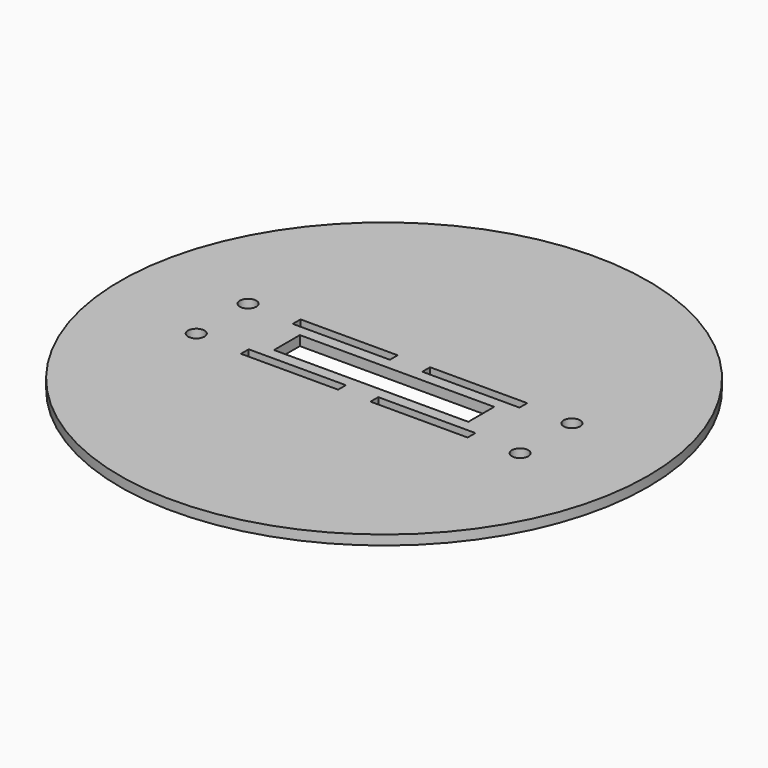
from build123d import *

# Parameters (mm, degrees)
F0_R     = 81.5
F0_R_2   = 2.55
F0_W     = 30
F0_H     = 3
F0_W_2   = 60
F0_H_2   = 10
F1_DEPTH = 3


# Not quite as in the source:
# - a feature names something its author has since deleted; it is built from what else it names


with BuildPart() as f1:
    # F0 (on Top) → F1 (new body)
    with BuildSketch(Plane.XY):
        Circle(F0_R)
        with Locations((-50, -10)):
            Circle(F0_R_2, mode=Mode.SUBTRACT)
        with Locations((-20, -10)):
            Rectangle(F0_W, F0_H, mode=Mode.SUBTRACT)
        with Locations((20, -10)):
            Rectangle(F0_W, F0_H, mode=Mode.SUBTRACT)
        with Locations((50, -10)):
            Circle(F0_R_2, mode=Mode.SUBTRACT)
        with Locations((-50, 10)):
            Circle(F0_R_2, mode=Mode.SUBTRACT)
        with Locations((-20, 10)):
            Rectangle(F0_W, F0_H, mode=Mode.SUBTRACT)
        Rectangle(F0_W_2, F0_H_2, mode=Mode.SUBTRACT)
        with Locations((20, 10)):
            Rectangle(F0_W, F0_H, mode=Mode.SUBTRACT)
        with Locations((50, 10)):
            Circle(F0_R_2, mode=Mode.SUBTRACT)
    extrude(amount=F1_DEPTH)


solid = f1.part
